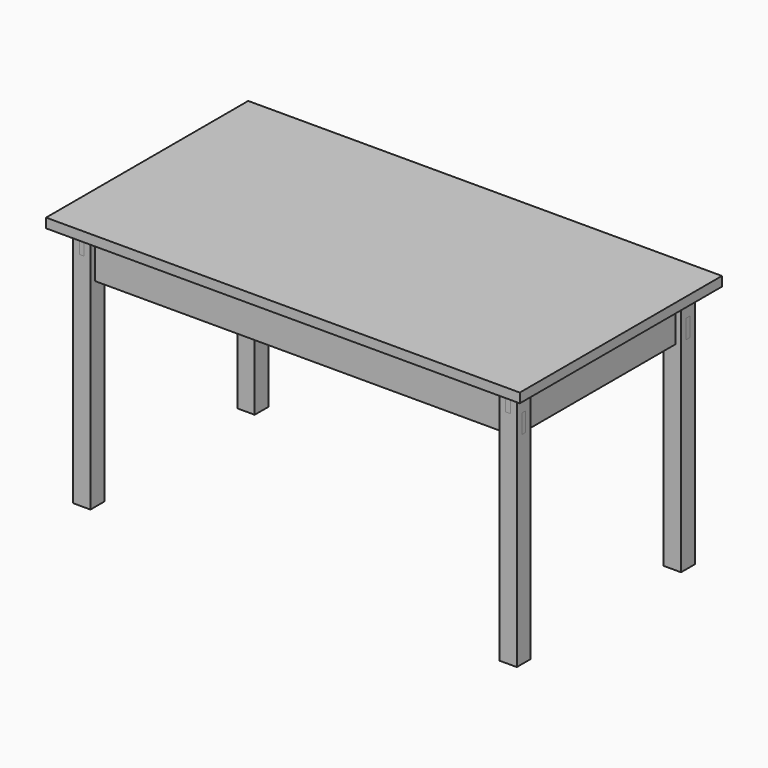
from build123d import *

# Parameters (mm, degrees)
F2_DEPTH  = 400
F10_DEPTH = 10
F4_W      = 55
F4_H      = 60
F11_DEPTH = 7.5
F12_DEPTH = 10
F13_DEPTH = 7.5
F14_DEPTH = 27.5
F9_W      = 15
F9_H      = 60
F15_DEPTH = 27.5
F16_COUNT = 2
F16_ANGLE = 180


with BuildPart() as f2:
    # F1 (on Front) → F2 (new body, symmetric)
    with BuildSketch(Plane.XZ):
        Polygon((750, 800), (-750, 800), (-750, 770), (-702.5, 770), (-647.5, 770), (647.5, 770), (750, 770), align=None)
    extrude(amount=F2_DEPTH, both=True)


with BuildPart() as f10:
    # F4 (on offset) → F10 (new body, symmetric)
    with BuildSketch(Plane.XZ.offset(325)):
        Polygon((647.5, 700), (647.5, 770), (-647.5, 770), (-647.5, 700), (-647.5, 640), (-647.5, 630), (647.5, 630), (647.5, 640), align=None)
    extrude(amount=F10_DEPTH, both=True)

    # F4 (on offset) → F11 (join, symmetric)
    with BuildSketch(Plane.XZ.offset(325)):
        with Locations((-675, 670)):
            Rectangle(F4_W, F4_H)
        with Locations((675, 670)):
            Rectangle(F4_W, F4_H)
    extrude(amount=F11_DEPTH, both=True)


with BuildPart() as f12:
    # F9 (on face) → F12 (new body, symmetric)
    with BuildSketch(Plane(origin=(-675, 0, 0), x_dir=(0, -1, 0), z_dir=(-1, 0, 0))):
        Polygon((-297.5, 630), (297.5, 630), (297.5, 700), (297.5, 770), (-297.5, 770), (-297.5, 700), align=None)
    extrude(amount=F12_DEPTH, both=True)

    # F6 (on offset) → F13 (join, symmetric)
    with BuildSketch(Plane(origin=(-675, 0, 0), x_dir=(0, -1, 0), z_dir=(-1, 0, 0))):
        Polygon((-297.5, 700), (-297.5, 770), (-335.7089757919, 770), (-335.9124362469, 770), (-352.5, 770), (-352.5, 700), (-332.5, 700), (-317.5, 700), align=None)
        Polygon((297.5, 700), (317.5, 700), (332.5, 700), (352.5, 700), (352.5, 770), (335.9124362469, 770), (335.7089757919, 770), (297.5, 770), align=None)
    extrude(amount=F13_DEPTH, both=True)


with BuildPart() as f14:
    # F8 (on face) → F14 (new body, symmetric)
    with BuildSketch(Plane.XZ.offset(325)):
        Polygon((-682.5, 770), (-702.5, 770), (-702.5, 0), (-647.5, 0), (-647.5, 630), (-647.5, 640), (-647.5, 700), (-647.5, 770), (-667.5, 770), (-667.5, 700), (-682.5, 700), align=None)
    extrude(amount=F14_DEPTH, both=True)

    # F9 (on face) → F15 (cut, symmetric)
    with BuildSketch(Plane(origin=(-675, 0, 0), x_dir=(0, -1, 0), z_dir=(-1, 0, 0))):
        with Locations((325, 670)):
            Rectangle(F9_W, F9_H)
    extrude(amount=F15_DEPTH, both=True, mode=Mode.SUBTRACT)


with BuildPart() as f16_1:
    # F16: instance of F10
    add(f10.part.rotate(Axis((0, 0, 400), (0, 0, 1)), 1 * F16_ANGLE / (F16_COUNT - 1)))


with BuildPart() as f16_2:
    # F16: instance of F14
    add(f14.part.rotate(Axis((0, 0, 400), (0, 0, 1)), 1 * F16_ANGLE / (F16_COUNT - 1)))


with BuildPart() as f17_1:
    # F17: instance of F14
    add(f14.part.mirror(Plane.XZ))


with BuildPart() as f18_1:
    # F18: instance of F12
    add(f12.part.mirror(Plane.YZ))


with BuildPart() as f18_2:
    # F18: instance of F14
    add(f14.part.mirror(Plane.YZ))


solid = Compound([f2.part, f10.part, f12.part, f14.part, f16_1.part, f16_2.part, f17_1.part, f18_1.part, f18_2.part])
